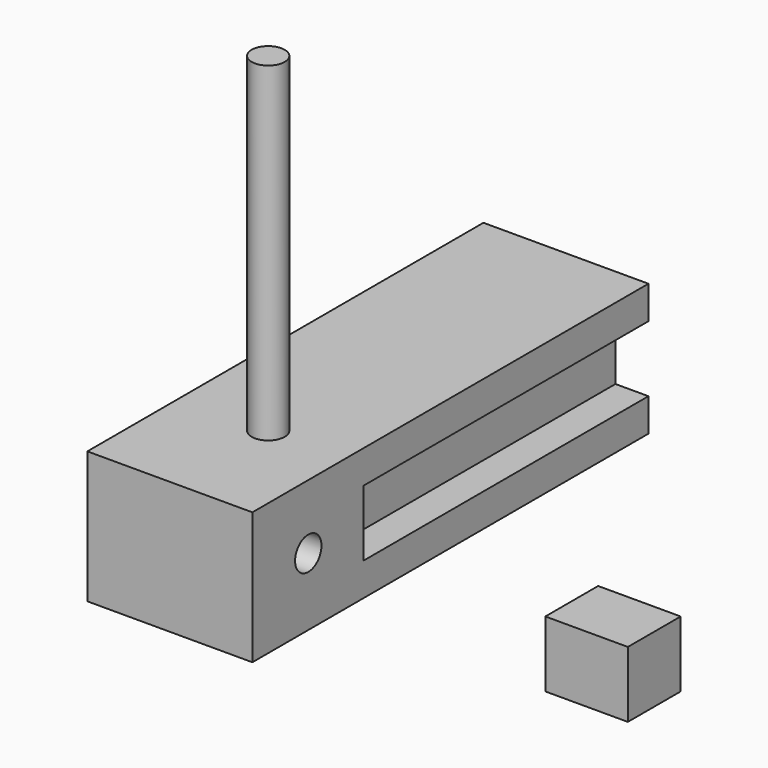
from build123d import *

# Parameters (mm, degrees)
F1_DEPTH  = 150
F2_W      = 20
F2_H      = 20
F3_DEPTH  = 25
F4_R      = 5
F5_DEPTH  = 15.2
F6_W      = 50
F6_H      = 40
F7_DEPTH  = 42
F8_R      = 5
F9_DEPTH  = 74.4
F10_R     = 5
F11_DEPTH = 100


# Not quite as in the source:
# - the program builds the solid bodies; features that only make, move or delete a surface that nothing else refers to are left out


with BuildPart() as f1:
    # F0 (on Front) → F1 (new body)
    with BuildSketch(Plane.XZ):
        Polygon((-16.1953240633, 25.6288190931), (-66.1953240633, 25.6288190931), (-66.1953240633, 15.6288190931), (-56.1953240633, 15.6288190931), (-56.1953240633, -4.3711809069), (-66.1953240633, -4.3711809069), (-66.1953240633, -14.3711809069), (-16.1953240633, -14.3711809069), (-16.1953240633, -4.3711809069), (-26.1953240633, -4.3711809069), (-26.1953240633, 15.6288190931), (-16.1953240633, 15.6288190931), align=None)
    extrude(amount=F1_DEPTH)

    # F6 (on face) → F7 (join)
    with BuildSketch(Plane.XZ.offset(150)):
        with Locations((-41.1953240633, 5.6288190931)):
            Rectangle(F6_W, F6_H)
    extrude(amount=-F7_DEPTH)

    # F8 (on Right) → F9 (cut)
    with BuildSketch(Plane.YZ):
        with Locations((-128.8177222013, 6.1109075323)):
            Circle(F8_R)
    extrude(amount=-F9_DEPTH, mode=Mode.SUBTRACT)


with BuildPart() as f3:
    # F2 (on Right) → F3 (new body)
    with BuildSketch(Plane.YZ):
        with Locations((-49.2914298177, -43.7528586388)):
            Rectangle(F2_W, F2_H)
    extrude(amount=F3_DEPTH)

    # F4 (on Right) → F5 (join)
    with BuildSketch(Plane.YZ):
        with Locations((-49.3974834681, -43.340831995)):
            Circle(F4_R)
    extrude(amount=F5_DEPTH)


with BuildPart() as f11:
    # F10 (on face) → F11 (new body)
    with BuildSketch(Plane.XY.offset(25.6288190931)):
        with Locations((-39.3799170852, -115.0251403451)):
            Circle(F10_R)
    extrude(amount=F11_DEPTH)


solid = Compound([f1.part, f3.part, f11.part])
